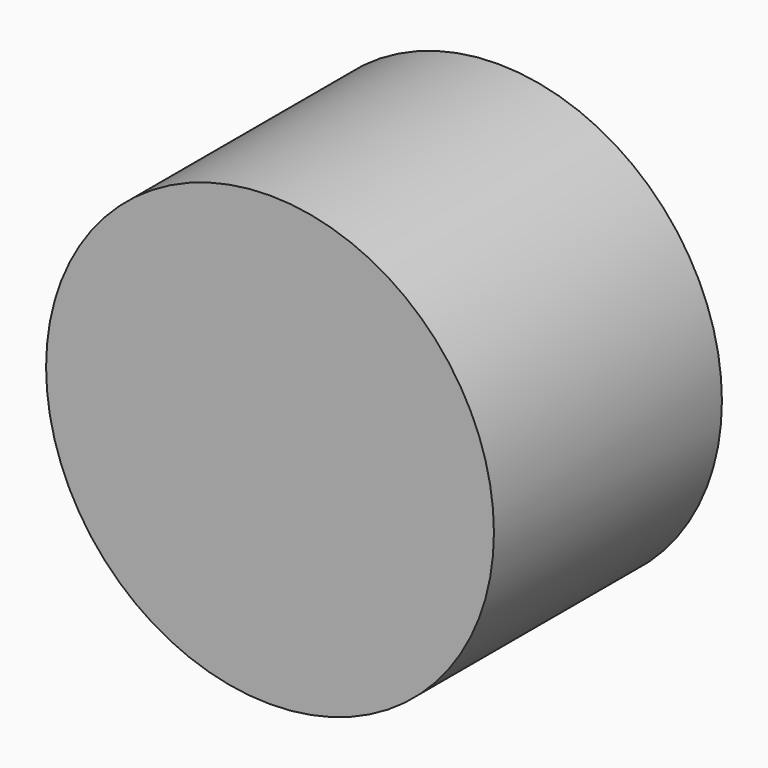
from build123d import *

# Parameters (mm, degrees)
F0_R     = 11
F1_DEPTH = 14


# Not quite as in the source:
# - a feature names something its author has since deleted; it is built from what else it names


with BuildPart() as f1:
    # F0 (on Front) → F1 (new body)
    with BuildSketch(Plane.XZ):
        Circle(F0_R)
    extrude(amount=-F1_DEPTH)


solid = f1.part
